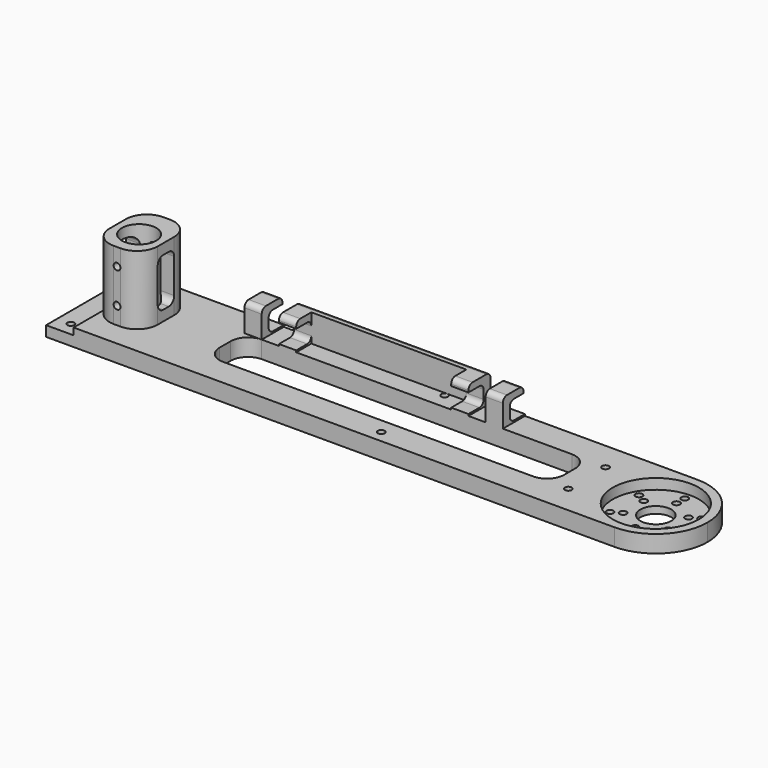
from build123d import *

# Parameters (mm, degrees)
F0_W          = 180
F0_H          = 30
F0_R          = 1
F0_W_2        = 100
F0_H_2        = 14
F1_DEPTH      = 5
F2_R          = 12.5
F2_R_2        = 1
F2_R_3        = 4.5
F3_DEPTH      = 3
F4_DEPTH      = 25
F5_R          = 14.99999
F2_R_4        = 5
F6_DEPTH      = 25
F7_R          = 5
F2_W          = 14
F2_H          = 18
F8_DEPTH      = 20
F9_R          = 6
F10_DEPTH     = 2
F11_W         = 6
F11_H         = 14
F12_DEPTH     = 25
F13_R         = 2
F15_DEPTH     = 25
F16_W         = 5
F16_H         = 8
F17_DEPTH     = 8
F18_W         = 5.5
F18_H         = 5.5
F19_W         = 5.5
F19_H         = 5.5
F20_W         = 5.5
F20_H         = 5.5
F21_W         = 5.5
F21_H         = 5.5
F22_DEPTH     = 6
F23_DEPTH     = 8
F24_DEPTH     = 0.5
F25_T1_DEPTH  = 5
F25_T3_DEPTH  = 5
F25_T5_DEPTH  = 5
F25_T7_DEPTH  = 5
F25_T9_DEPTH  = 12.5
F25_T11_DEPTH = 8.75
F25_T13_DEPTH = 12.5
F25_T15_DEPTH = 8.75
F25_T17_DEPTH = 12.5
F25_T19_DEPTH = 12.5
F25_T21_DEPTH = 45


# Not quite as in the source:
# - a fillet or chamfer that OpenCascade refuses, or shapes differently, is made with other operations: its cross-section is extruded or revolved along the edge and cut away or added
# - a fillet or chamfer is up to 0.001 mm smaller than in the source, because OpenCascade refuses the exact size
# - a feature names something its author has since deleted; it is built from what else it names


with BuildPart() as f1:
    # F0 (on Top) → F1 (new body)
    with BuildSketch(Plane.XY):
        with Locations((10, -11.8972941886)):
            Rectangle(F0_W, F0_H)
        with Locations((-76, -22.8972941886)):
            Circle(F0_R, mode=Mode.SUBTRACT)
        with Locations((14.5, -23.3972941886)):
            Circle(F0_R, mode=Mode.SUBTRACT)
        with Locations((10, -11.8972941886)):
            Rectangle(F0_W_2, F0_H_2, mode=Mode.SUBTRACT)
        with Locations((65, -18.6472941886)):
            Circle(F0_R, mode=Mode.SUBTRACT)
        with Locations((-76, -0.8972941886)):
            Circle(F0_R, mode=Mode.SUBTRACT)
        with Locations((65, -5.1472941886)):
            Circle(F0_R, mode=Mode.SUBTRACT)
        with Locations((14.5, -0.3972941886)):
            Circle(F0_R, mode=Mode.SUBTRACT)
    extrude(amount=F1_DEPTH)

    # F2 (on face) → F3 (cut)
    with BuildSketch(Plane.XY.offset(5)):
        with Locations((85, -11.8972941886)):
            Circle(F2_R)
        with Locations((85, -22.3972941886)):
            Circle(F2_R_2, mode=Mode.SUBTRACT)
        with Locations((85, -19.3972941886)):
            Circle(F2_R_2, mode=Mode.SUBTRACT)
        with Locations((75.9067332603, -17.1472941886)):
            Circle(F2_R_2, mode=Mode.SUBTRACT)
        with Locations((78.5048094716, -15.6472941886)):
            Circle(F2_R_2, mode=Mode.SUBTRACT)
        with Locations((94.0932667397, -17.1472941886)):
            Circle(F2_R_2, mode=Mode.SUBTRACT)
        with Locations((91.4951905284, -15.6472941886)):
            Circle(F2_R_2, mode=Mode.SUBTRACT)
        with Locations((85, -11.8972941886)):
            Circle(F2_R_3, mode=Mode.SUBTRACT)
        with Locations((78.5048094716, -8.1472941886)):
            Circle(F2_R_2, mode=Mode.SUBTRACT)
        with Locations((91.4951905284, -8.1472941886)):
            Circle(F2_R_2, mode=Mode.SUBTRACT)
        with Locations((75.9067332603, -6.6472941886)):
            Circle(F2_R_2, mode=Mode.SUBTRACT)
        with Locations((94.0932667397, -6.6472941886)):
            Circle(F2_R_2, mode=Mode.SUBTRACT)
        with Locations((85, -4.3972941886)):
            Circle(F2_R_2, mode=Mode.SUBTRACT)
        with Locations((85, -1.3972941886)):
            Circle(F2_R_2, mode=Mode.SUBTRACT)
    extrude(amount=-F3_DEPTH, mode=Mode.SUBTRACT)

    # F2 (on face) → F4 (cut)
    with BuildSketch(Plane.XY.offset(5)):
        with Locations((85, -11.8972941886)):
            Circle(F2_R_3)
        with Locations((85, -4.3972941886)):
            Circle(F2_R_2)
        with Locations((85, -19.3972941886)):
            Circle(F2_R_2)
        with Locations((91.4951905284, -8.1472941886)):
            Circle(F2_R_2)
        with Locations((91.4951905284, -15.6472941886)):
            Circle(F2_R_2)
        with Locations((78.5048094716, -15.6472941886)):
            Circle(F2_R_2)
        with Locations((78.5048094716, -8.1472941886)):
            Circle(F2_R_2)
        with Locations((85, -1.3972941886)):
            Circle(F2_R_2)
        with Locations((75.9067332603, -6.6472941886)):
            Circle(F2_R_2)
        with Locations((75.9067332603, -17.1472941886)):
            Circle(F2_R_2)
        with Locations((85, -22.3972941886)):
            Circle(F2_R_2)
        with Locations((94.0932667397, -17.1472941886)):
            Circle(F2_R_2)
        with Locations((94.0932667397, -6.6472941886)):
            Circle(F2_R_2)
    extrude(amount=-F4_DEPTH, mode=Mode.SUBTRACT)

    # F5 (radius 15 in the source; OpenCascade refuses exactly that, so slightly less here)
    f5_edges = [f1.edges().sort_by_distance(p)[0] for p in [
        (100, 3.102706, 2.5),
        (100, -26.897294, 2.5),
    ]]
    fillet(f5_edges, radius=F5_R)

    # F2 (on face) → F6 (cut)
    with BuildSketch(Plane.XY.offset(5)):
        with Locations((-65, -11.8972941886)):
            Circle(F2_R_4)
    extrude(amount=-F6_DEPTH, mode=Mode.SUBTRACT)

    # F7
    f7_edges = [f1.edges().sort_by_distance(p)[0] for p in [
        (-40, -4.897294, 2.5),
        (-40, -18.897294, 2.5),
        (60, -4.897294, 2.5),
        (60, -18.897294, 2.5),
    ]]
    fillet(f7_edges, radius=F7_R)

    # F2 (on face) → F8 (join)
    with BuildSketch(Plane.XY.offset(5)):
        with Locations((-65, -10.8972941886)):
            Rectangle(F2_W, F2_H)
        with Locations((-65, -11.8972941886)):
            Circle(F2_R_4, mode=Mode.SUBTRACT)
    extrude(amount=F8_DEPTH)

    # F9
    f9_edges = [f1.edges().sort_by_distance(p)[0] for p in [
        (-72, -19.897294, 15),
        (-58, -19.897294, 15),
        (-72, -1.897294, 15),
        (-58, -1.897294, 15),
    ]]
    fillet(f9_edges, radius=F9_R)

    # F2 (on face) → F10 (cut)
    with BuildSketch(Plane.XY.offset(5)):
        Polygon((-72, -19.8972941886), (-72, -1.8972941886), (-72, 3.1027058114), (-80, 3.1027058114), (-80, -26.8972941886), (-72, -26.8972941886), align=None)
        with Locations((-76, -22.8972941886)):
            Circle(F2_R_2, mode=Mode.SUBTRACT)
        with Locations((-76, -0.8972941886)):
            Circle(F2_R_2, mode=Mode.SUBTRACT)
    extrude(amount=-F10_DEPTH, mode=Mode.SUBTRACT)

    # F11 (on face) → F12 (cut)
    with BuildSketch(Plane.YZ.offset(-58)):
        with Locations((-10.8972941886, 15)):
            Rectangle(F11_W, F11_H)
    extrude(amount=-F12_DEPTH, mode=Mode.SUBTRACT)

    # F13
    f13_edges = [f1.edges().sort_by_distance(p)[0] for p in [
        (-59.208712, -13.897294, 8),
        (-60, -7.897294, 8),
        (-60, -7.897294, 22),
        (-59.208712, -13.897294, 22),
        (-70.791288, -13.897294, 8),
        (-70, -7.897294, 8),
        (-70, -7.897294, 22),
        (-70.791288, -13.897294, 22),
    ]]
    fillet(f13_edges, radius=F13_R)

    # F14 (on face) → F15 (cut)
    with BuildSketch(Plane(origin=(0, -1.8972941886, 0), x_dir=(-1, 0, 0), z_dir=(0, 1, 0))):
        with BuildLine():
            ThreePointArc((64, 20), (65, 19), (66, 20))
            ThreePointArc((66, 20), (65, 21), (64, 20))
        make_face()
        with BuildLine():
            ThreePointArc((64, 10), (65, 9), (66, 10))
            ThreePointArc((66, 10), (65, 11), (64, 10))
        make_face()
    extrude(amount=-F15_DEPTH, mode=Mode.SUBTRACT)

    # F16 (on face) → F17 (join)
    with BuildSketch(Plane.XY.offset(5)):
        with Locations((-37.5, -0.8972941886)):
            Rectangle(F16_W, F16_H)
        Polygon((-25, 3.1027058114), (-30, 3.1027058114), (-30, -4.8972941886), (-25, -4.8972941886), (-25, 0.6027058114), align=None)
        Polygon((25, 3.1027058114), (20, 3.1027058114), (20, 0.6027058114), (20, -4.8972941886), (25, -4.8972941886), align=None)
        with Locations((32.5, -0.8972941886)):
            Rectangle(F16_W, F16_H)
    extrude(amount=F17_DEPTH)

    # F18 (on face) + F19 (on face) + F20 (on face) + F21 (on face) → F22 (cut)
    with BuildSketch(Plane(origin=(-40, 0, 0), x_dir=(0, -1, 0), z_dir=(-1, 0, 0))):
        with Locations((-0.3527058114, 8.25)):
            Rectangle(F18_W, F18_H)
    with BuildSketch(Plane(origin=(-30, 0, 0), x_dir=(0, -1, 0), z_dir=(-1, 0, 0))):
        with Locations((2.1472941886, 8.25)):
            Rectangle(F19_W, F19_H)
    with BuildSketch(Plane(origin=(20, 0, 0), x_dir=(0, -1, 0), z_dir=(-1, 0, 0))):
        with Locations((2.1472941886, 8.25)):
            Rectangle(F20_W, F20_H)
    with BuildSketch(Plane(origin=(30, 0, 0), x_dir=(0, -1, 0), z_dir=(-1, 0, 0))):
        with Locations((-0.3527058114, 8.25)):
            Rectangle(F21_W, F21_H)
    extrude(amount=-F22_DEPTH, mode=Mode.SUBTRACT)

    # F16 (on face) → F23 (join)
    with BuildSketch(Plane.XY.offset(5)):
        Polygon((20, 3.1027058114), (-25, 3.1027058114), (-25, 0.6027058114), (14.5000000057, 0.6027058114), (20, 0.6027058114), align=None)
    extrude(amount=F23_DEPTH)

    # F24 (cut): faces of the model
    f24_faces = [f1.faces().sort_by_distance(p)[0] for p in [
        (32.5, 3.1027058114, 12),
        (22.5, -4.8972941886, 12),
        (-27.5, -4.8972941886, 12),
        (-37.5, 3.1027058114, 12),
    ]]
    extrude(f24_faces, amount=-F24_DEPTH, dir=(0, 1, 0), mode=Mode.SUBTRACT)

    # F25: fillet of radius 1.5 on 16 edges, made by hand

    # F25_s2 → F25_t1 (join)
    with BuildSketch(Plane.YZ.offset(30)):
        with BuildLine():
            ThreePointArc((-2.3972941886, 9.5), (-1.9579543604, 10.5606601718), (-0.8972941886, 11))
            Line((-0.8972941886, 11), (-2.3972941886, 11))
            Line((-2.3972941886, 11), (-2.3972941886, 9.5))
        make_face()
        with BuildLine():
            ThreePointArc((-0.8972941886, 5.5), (-1.9579543604, 5.9393398282), (-2.3972941886, 7))
            Line((-2.3972941886, 7), (-2.3972941886, 5.5))
            Line((-2.3972941886, 5.5), (-0.8972941886, 5.5))
        make_face()
    extrude(amount=F25_T1_DEPTH)

    # F25_s4 → F25_t3 (join)
    with BuildSketch(Plane.YZ.offset(-40)):
        with BuildLine():
            ThreePointArc((-2.3972941886, 7), (-1.9579543604, 5.9393398282), (-0.8972941886, 5.5))
            Line((-0.8972941886, 5.5), (-2.3972941886, 5.5))
            Line((-2.3972941886, 5.5), (-2.3972941886, 7))
        make_face()
        with BuildLine():
            ThreePointArc((-0.8972941886, 11), (-1.9579543604, 10.5606601718), (-2.3972941886, 9.5))
            Line((-2.3972941886, 9.5), (-2.3972941886, 11))
            Line((-2.3972941886, 11), (-0.8972941886, 11))
        make_face()
    extrude(amount=F25_T3_DEPTH)

    # F25_s6 → F25_t5 (join)
    with BuildSketch(Plane.YZ.offset(-30)):
        with BuildLine():
            ThreePointArc((-0.8972941886, 5.5), (0.1633659832, 5.9393398282), (0.6027058114, 7))
            Line((0.6027058114, 7), (0.6027058114, 5.5))
            Line((0.6027058114, 5.5), (-0.8972941886, 5.5))
        make_face()
        with BuildLine():
            ThreePointArc((0.6027058114, 9.5), (0.1633659832, 10.5606601718), (-0.8972941886, 11))
            Line((-0.8972941886, 11), (0.6027058114, 11))
            Line((0.6027058114, 11), (0.6027058114, 9.5))
        make_face()
    extrude(amount=F25_T5_DEPTH)

    # F25_s8 → F25_t7 (join)
    with BuildSketch(Plane.YZ.offset(20)):
        with BuildLine():
            ThreePointArc((-0.8972941886, 5.5), (0.1633659832, 5.9393398282), (0.6027058114, 7))
            Line((0.6027058114, 7), (0.6027058114, 5.5))
            Line((0.6027058114, 5.5), (-0.8972941886, 5.5))
        make_face()
        with BuildLine():
            ThreePointArc((-0.8972941886, 11), (0.1633659832, 10.5606601718), (0.6027058114, 9.5))
            Line((0.6027058114, 9.5), (0.6027058114, 11))
            Line((0.6027058114, 11), (-0.8972941886, 11))
        make_face()
    extrude(amount=F25_T7_DEPTH)

    # F25_s10 → F25_t9 (cut)
    with BuildSketch(Plane.YZ.offset(-43.75)):
        with BuildLine():
            ThreePointArc((1.1027058114, 13), (2.1633659832, 12.5606601718), (2.6027058114, 11.5))
            Line((2.6027058114, 11.5), (2.6027058114, 13))
            Line((2.6027058114, 13), (1.1027058114, 13))
        make_face()
        with BuildLine():
            ThreePointArc((-4.8972941886, 11.5), (-4.4579543604, 12.5606601718), (-3.3972941886, 13))
            Line((-3.3972941886, 13), (-4.8972941886, 13))
            Line((-4.8972941886, 13), (-4.8972941886, 11.5))
        make_face()
    extrude(amount=F25_T9_DEPTH, mode=Mode.SUBTRACT)

    # F25_s12 → F25_t11 (cut)
    with BuildSketch(Plane.YZ.offset(-33.75)):
        with BuildLine():
            ThreePointArc((3.1027058114, 11.5), (2.6633659832, 12.5606601718), (1.6027058114, 13))
            Line((1.6027058114, 13), (3.1027058114, 13))
            Line((3.1027058114, 13), (3.1027058114, 11.5))
        make_face()
    extrude(amount=F25_T11_DEPTH, mode=Mode.SUBTRACT)

    # F25_s14 → F25_t13 (cut)
    with BuildSketch(Plane.YZ.offset(-33.75)):
        with BuildLine():
            ThreePointArc((-3.3972941886, 13), (-4.4579543604, 12.5606601718), (-4.8972941886, 11.5))
            Line((-4.8972941886, 11.5), (-4.8972941886, 13))
            Line((-4.8972941886, 13), (-3.3972941886, 13))
        make_face()
    extrude(amount=F25_T13_DEPTH, mode=Mode.SUBTRACT)

    # F25_s16 → F25_t15 (cut)
    with BuildSketch(Plane.YZ.offset(20)):
        with BuildLine():
            ThreePointArc((3.1027058114, 11.5), (2.6633659832, 12.5606601718), (1.6027058114, 13))
            Line((1.6027058114, 13), (3.1027058114, 13))
            Line((3.1027058114, 13), (3.1027058114, 11.5))
        make_face()
    extrude(amount=F25_T15_DEPTH, mode=Mode.SUBTRACT)

    # F25_s18 → F25_t17 (cut)
    with BuildSketch(Plane.YZ.offset(16.25)):
        with BuildLine():
            ThreePointArc((-3.3972941886, 13), (-4.4579543604, 12.5606601718), (-4.8972941886, 11.5))
            Line((-4.8972941886, 11.5), (-4.8972941886, 13))
            Line((-4.8972941886, 13), (-3.3972941886, 13))
        make_face()
    extrude(amount=F25_T17_DEPTH, mode=Mode.SUBTRACT)

    # F25_s20 → F25_t19 (cut)
    with BuildSketch(Plane.YZ.offset(26.25)):
        with BuildLine():
            ThreePointArc((2.6027058114, 11.5), (2.1633659832, 12.5606601718), (1.1027058114, 13))
            Line((1.1027058114, 13), (2.6027058114, 13))
            Line((2.6027058114, 13), (2.6027058114, 11.5))
        make_face()
        with BuildLine():
            ThreePointArc((-4.8972941886, 11.5), (-4.4579543604, 12.5606601718), (-3.3972941886, 13))
            Line((-3.3972941886, 13), (-4.8972941886, 13))
            Line((-4.8972941886, 13), (-4.8972941886, 11.5))
        make_face()
    extrude(amount=F25_T19_DEPTH, mode=Mode.SUBTRACT)

    # F25_s22 → F25_t21 (cut)
    with BuildSketch(Plane.YZ.offset(-25)):
        with BuildLine():
            ThreePointArc((3.1027058114, 11.5), (2.6633659832, 12.5606601718), (1.6027058114, 13))
            Line((1.6027058114, 13), (3.1027058114, 13))
            Line((3.1027058114, 13), (3.1027058114, 11.5))
        make_face()
    extrude(amount=F25_T21_DEPTH, mode=Mode.SUBTRACT)


solid = f1.part
